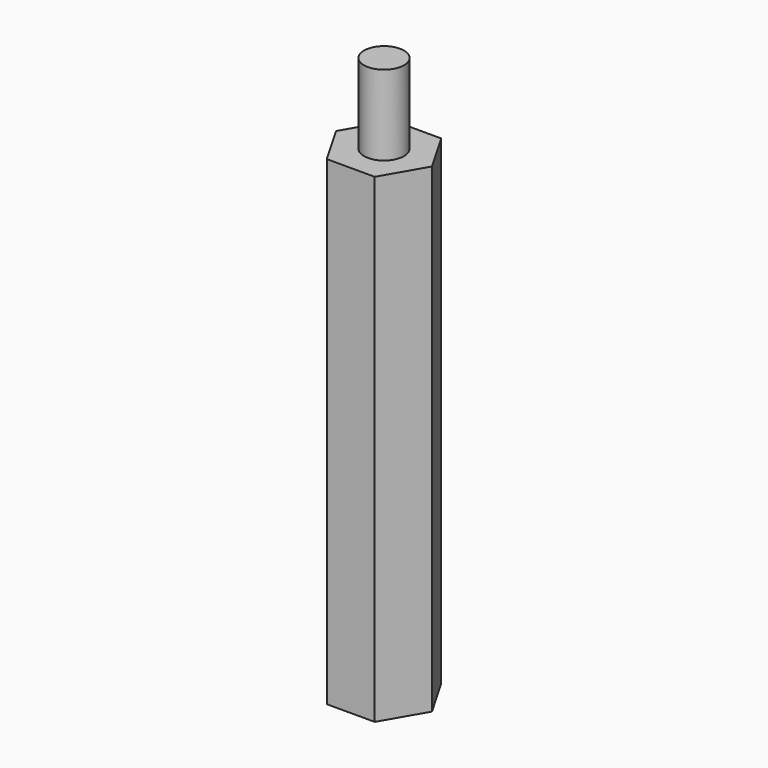
from build123d import *

# Parameters (mm, degrees)
F0_R     = 1.25
F1_DEPTH = 30
F2_DEPTH = 35
F3_R     = 1.25
F4_DEPTH = 28


# Not quite as in the source:
# - a feature names something its author has since deleted; it is built from what else it names


with BuildPart() as f1:
    # F0 (on Top) → F1 (new body)
    with BuildSketch(Plane.XY):
        Polygon((1.5, 2.5980762114), (-1.5, 2.5980762114), (-3, 0), (-1.5, -2.5980762114), (1.5, -2.5980762114), (3, 0), align=None)
        Circle(F0_R, mode=Mode.SUBTRACT)
    extrude(amount=F1_DEPTH)

    # F0 (on Top) → F2 (join)
    with BuildSketch(Plane.XY):
        Circle(F0_R)
    extrude(amount=F2_DEPTH)

    # F3 (on face) → F4 (cut)
    with BuildSketch(Plane(origin=(0, 0, 0), x_dir=(1, 0, 0), z_dir=(0, 0, -1))):
        Circle(F3_R)
    extrude(amount=-F4_DEPTH, mode=Mode.SUBTRACT)


solid = f1.part
